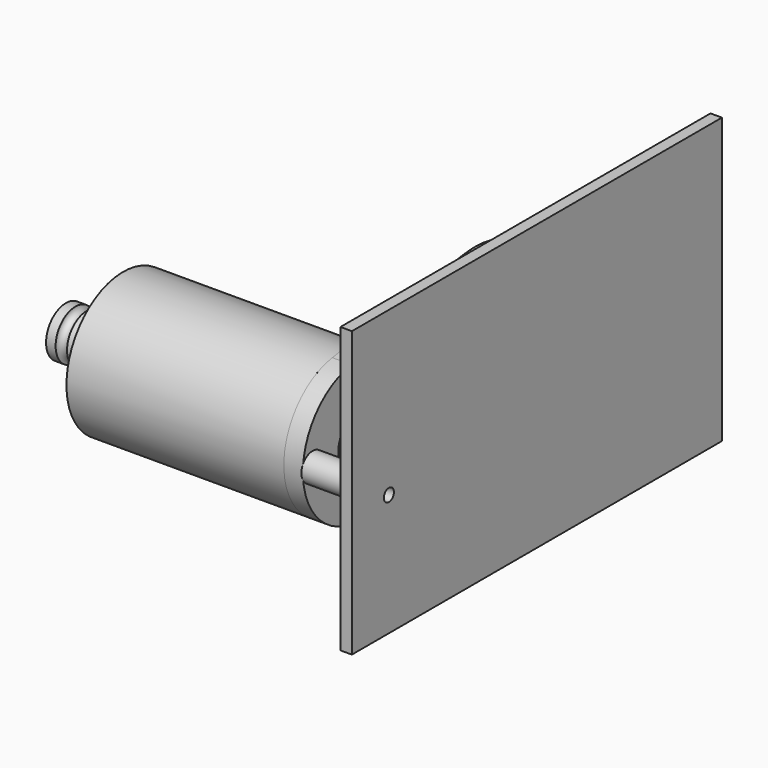
from build123d import *

# Parameters (mm, degrees)
F0_R      = 18.6
F1_DEPTH  = 57
F2_R      = 6.5
F3_DEPTH  = 4.4
F4_R      = 4.8
F5_DEPTH  = 8.8
F6_R      = 18.6
F6_R_2    = 7
F7_DEPTH  = 5
F8_R      = 25
F8_R_2    = 16.5
F9_DEPTH  = 5
F11_R     = 16.5
F12_DEPTH = 5
F13_R     = 1.5
F14_DEPTH = 25
F15_R     = 1.5
F16_DEPTH = 25
F20_R     = 3.7280937336
F20_R_2   = 1.65
F21_DEPTH = 20
F20_R_3   = 3.440231923
F20_R_4   = 3.7779559
F20_R_5   = 3.6823688958
F22_W     = 121.2965659797
F22_H     = 74.6714472771
F22_R     = 3.6823688958
F23_DEPTH = 3


with BuildPart() as f1:
    # F0 (on Right) → F1 (new body)
    with BuildSketch(Plane.YZ):
        Circle(F0_R)
    extrude(amount=F1_DEPTH)

    # F2 (on face) → F3 (join)
    with BuildSketch(Plane.YZ.offset(57)):
        Circle(F2_R)
    extrude(amount=F3_DEPTH)

    # F4 (on face) → F5 (join)
    with BuildSketch(Plane.YZ.offset(61.4)):
        Circle(F4_R)
    extrude(amount=F5_DEPTH)


with BuildPart() as f7:
    # F6 (on face) → F7 (new body)
    with BuildSketch(Plane.YZ.offset(57)):
        Circle(F6_R)
        Circle(F6_R_2, mode=Mode.SUBTRACT)
    extrude(amount=F7_DEPTH)

    # F11 (on face) → F12 (join)
    with BuildSketch(Plane.YZ.offset(62)):
        with BuildLine():
            Line((40.3636363636, 24.7341233826), (-2.7054545455, 18.4021877966))
            ThreePointArc((-2.7054545455, 18.4021877966), (12.1580949465, 14.0762469172), (18.6, 0))
            ThreePointArc((18.6, 0), (12.1580949465, -14.0762469172), (-2.7054545455, -18.4021877966))
            Line((-2.7054545455, -18.4021877966), (40.3636363636, -24.7341233826))
            ThreePointArc((40.3636363636, -24.7341233826), (69, 0), (40.3636363636, 24.7341233826))
        make_face()
        with Locations((44, 0)):
            Circle(F11_R, mode=Mode.SUBTRACT)
    extrude(amount=-F12_DEPTH)

    # F13 (on face) → F14 (cut)
    with BuildSketch(Plane.YZ.offset(62)):
        with Locations((0, 12.5)):
            Circle(F13_R)
        with Locations((0, -12.5)):
            Circle(F13_R)
    extrude(amount=-F14_DEPTH, mode=Mode.SUBTRACT)

    # F15 (on face) → F16 (cut)
    with BuildSketch(Plane.YZ.offset(62)):
        with Locations((23, 0)):
            Circle(F15_R)
        with Locations((43.3874823415, 20.9910652926)):
            Circle(F15_R)
        with Locations((65, 0)):
            Circle(F15_R)
        with Locations((43.4260752234, -20.9921559243)):
            Circle(F15_R)
    extrude(amount=-F16_DEPTH, mode=Mode.SUBTRACT)


with BuildPart() as f9:
    # F8 (on face) → F9 (new body)
    with BuildSketch(Plane.YZ.offset(62)):
        with Locations((45, 0)):
            Circle(F8_R)
        with Locations((45, 0)):
            Circle(F8_R_2, mode=Mode.SUBTRACT)
    extrude(amount=-F9_DEPTH)


with BuildPart() as f18:
    # F17 (on Front) → F18 (revolve)
    with BuildSketch(Plane.XZ):
        with BuildLine():
            Line((-15.0285773807, 6.5), (-15.0285773807, 4))
            Line((-15.0285773807, 4), (-7.0285773807, 4))
            Line((-7.0285773807, 4), (-7.0285773807, 6.5))
            Line((-7.0285773807, 6.5), (-9.5285773807, 6.5))
            ThreePointArc((-9.5285773807, 6.5), (-11.0285773807, 5), (-12.5285773807, 6.5))
            Line((-12.5285773807, 6.5), (-15.0285773807, 6.5))
        make_face()
    revolve(axis=Axis((-10.1703209803, 0, 0), (-1, 0, 0)))


with BuildPart() as f21:
    # F20 (on face) → F21 (new body)
    with BuildSketch(Plane.YZ.offset(62)):
        with Locations((26.2333868136, 17.169676806)):
            Circle(F20_R)
        with Locations((26.2333868136, 17.169676806)):
            Circle(F20_R_2, mode=Mode.SUBTRACT)
    extrude(amount=F21_DEPTH)



with BuildPart() as f21b:
    # F20 (on face) → F21, piece 2 (new body)
    with BuildSketch(Plane.YZ.offset(62)):
        with Locations((59.1149660932, -14.1026837679)):
            Circle(F20_R_3)
        with Locations((59.1149660932, -14.1026837679)):
            Circle(F20_R_2, mode=Mode.SUBTRACT)
    extrude(amount=F21_DEPTH)


with BuildPart() as f21c:
    # F20 (on face) → F21, piece 3 (new body)
    with BuildSketch(Plane.YZ.offset(62)):
        with Locations((18.3423645794, -17.7443698049)):
            Circle(F20_R_4)
        with Locations((18.3423645794, -17.7443698049)):
            Circle(F20_R_2, mode=Mode.SUBTRACT)
    extrude(amount=F21_DEPTH)


with BuildPart() as f21d:
    # F20 (on face) → F21, piece 4 (new body)
    with BuildSketch(Plane.YZ.offset(62)):
        with Locations((-15.4150349557, 0)):
            Circle(F20_R_5)
        with Locations((-15.4150349557, 0)):
            Circle(F20_R_2, mode=Mode.SUBTRACT)
    extrude(amount=F21_DEPTH)


with BuildPart() as f21_1:
    add(f21.part)

    add(f21b.part)  # F23 merges F21b

    add(f21c.part)  # F23 merges F21c

    add(f21d.part)  # F23 merges F21d
    # F22 (on face) → F23 (join)
    with BuildSketch(Plane.YZ.offset(82)):
        with Locations((33.1084076315, 5.4097175598)):
            Rectangle(F22_W, F22_H)
        with Locations((-15.4150349557, 0)):
            Circle(F22_R, mode=Mode.SUBTRACT)
    extrude(amount=-F23_DEPTH)


solid = Compound([f1.part, f7.part, f18.part, f21_1.part])
